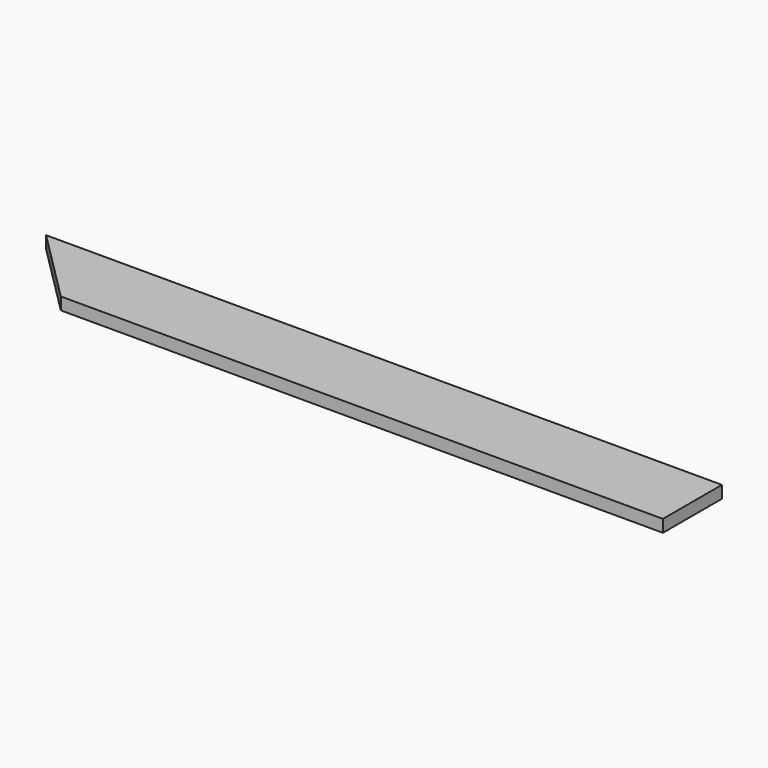
from build123d import *

# Parameters (mm, degrees)
F0_W     = 1397
F0_H     = 152.4
F1_DEPTH = 25.4
F2_SIZE  = 152.39999


# Not quite as in the source:
# - a fillet or chamfer is up to 0.001 mm smaller than in the source, because OpenCascade refuses the exact size


with BuildPart() as f1:
    # F0 (on Top) → F1 (new body)
    with BuildSketch(Plane.XY):
        with Locations((698.5, -76.2)):
            Rectangle(F0_W, F0_H)
    extrude(amount=F1_DEPTH)

    # F2 (size 152.4 in the source; OpenCascade refuses exactly that, so slightly less here)
    f2_edges = [f1.edges().sort_by_distance(p)[0] for p in [
        (0, -152.4, 12.7),
    ]]
    chamfer(f2_edges, length=F2_SIZE)


solid = f1.part
